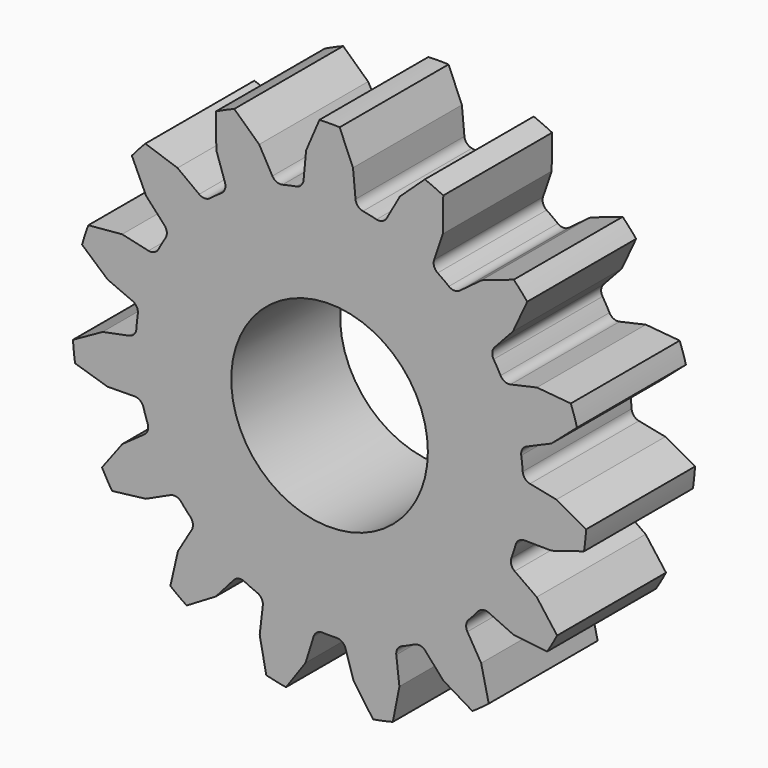
from build123d import *

# Parameters (mm, degrees)
F0_R     = 3.25
F1_DEPTH = 4.5


# Not quite as in the source:
# - ends of sketch curves that miss each other by under 0.0002 mm in the source are joined


with BuildPart() as f1:
    # F0 (on Front) → F1 (new body)
    with BuildSketch(Plane.XZ):
        with BuildLine():
            ThreePointArc((-6.3848473051, 0.378745021), (-6.458741388, 0.201395137), (-6.6250810223, 0.1052471112))
            Line((-6.6250810223, 0.1052471112), (-7.499995, -0.070416))
            Line((-7.499995, -0.070416), (-8.481787, -0.617539))
            ThreePointArc((-8.481787, -0.617539), (-8.4534361937, -0.9498951475), (-8.4120672698, -1.2808810391))
            Line((-8.4120672698, -1.2808810391), (-7.337975, -1.611925))
            Line((-7.337975, -1.611925), (-6.445659, -1.601845))
            ThreePointArc((-6.445659, -1.601845), (-6.2629631412, -1.6613077046), (-6.1538101366, -1.819419039))
            ThreePointArc((-6.1538101366, -1.819419039), (-6.0867618577, -2.039112292), (-6.0118718389, -2.2562609412))
            ThreePointArc((-6.0118718389, -2.2562609412), (-6.0072434399, -2.4483319562), (-6.120095855, -2.6038242044))
            Line((-6.120095855, -2.6038242044), (-6.84792, -3.12016))
            Line((-6.84792, -3.12016), (-7.522298, -4.019312))
            ThreePointArc((-7.522298, -4.019312), (-7.3612165371, -4.3114029523), (-7.1888002117, -4.5969471336))
            Line((-7.1888002117, -4.5969471336), (-6.07292, -4.462499))
            Line((-6.07292, -4.462499), (-5.261849, -4.090353))
            ThreePointArc((-5.261849, -4.090353), (-5.0707630565, -4.0703658396), (-4.9067374821, -4.1704104038))
            ThreePointArc((-4.9067374821, -4.1704104038), (-4.7561274158, -4.343839289), (-4.5993898038, -4.5117538102))
            ThreePointArc((-4.5993898038, -4.5117538102), (-4.5170386347, -4.6853377004), (-4.5568904277, -4.8732883391))
            Line((-4.5568904277, -4.8732883391), (-5.011778, -5.641017))
            Line((-5.011778, -5.641017), (-5.262135, -6.736727))
            ThreePointArc((-5.262135, -6.736727), (-4.9961722078, -6.9380502226), (-4.7225170454, -7.128782068))
            Line((-4.7225170454, -7.128782068), (-3.757802, -6.552084))
            Line((-3.757802, -6.552084), (-3.168217, -5.882218))
            ThreePointArc((-3.168217, -5.882218), (-3.0017803181, -5.7862379026), (-2.8112432041, -5.8109184175))
            ThreePointArc((-2.8112432041, -5.8109184175), (-2.6031126369, -5.9080957654), (-2.3916319825, -5.9977409564))
            ThreePointArc((-2.3916319825, -5.9977409564), (-2.2457975094, -6.1228225948), (-2.2057577098, -6.3107329173))
            Line((-2.2057577098, -6.3107329173), (-2.309055, -7.197108))
            Line((-2.309055, -7.197108), (-2.092101, -8.299918))
            ThreePointArc((-2.092101, -8.299918), (-1.7672462291, -8.3756592743), (-1.4396719873, -8.4385959262))
            Line((-1.4396719873, -8.4385959262), (-0.792926, -7.519371))
            Line((-0.792926, -7.519371), (-0.526772, -6.667613))
            ThreePointArc((-0.526772, -6.667613), (-0.4137637804, -6.5122339125), (-0.2296610073, -6.457282204))
            ThreePointArc((-0.2296610073, -6.457282204), (2.4984e-06, -6.461404), (0.229662, -6.457281998))
            ThreePointArc((0.229662, -6.457281998), (0.4137637804, -6.5122339125), (0.5267720218, -6.6676129932))
            Line((0.5267720218, -6.6676129932), (0.792926, -7.519371))
            Line((0.792926, -7.519371), (1.439676, -8.438595))
            ThreePointArc((1.439676, -8.438595), (1.7672522889, -8.3756579862), (2.0921050032, -8.2999170124))
            Line((2.0921050032, -8.2999170124), (2.309055, -7.197108))
            Line((2.309055, -7.197108), (2.205757, -6.310733))
            ThreePointArc((2.205757, -6.310733), (2.2457975094, -6.1228225948), (2.3916327595, -5.9977404031))
            ThreePointArc((2.3916327595, -5.9977404031), (2.6031159206, -5.9080943034), (2.8112438605, -5.8109177148))
            ThreePointArc((2.8112438605, -5.8109177148), (3.0017803181, -5.7862379026), (3.1682168748, -5.8822191102))
            Line((3.1682168748, -5.8822191102), (3.757802, -6.552084))
            Line((3.757802, -6.552084), (4.72252, -7.12878))
            ThreePointArc((4.72252, -7.12878), (4.9961769033, -6.9380468111), (5.2621377529, -6.7367246866))
            Line((5.2621377529, -6.7367246866), (5.011778, -5.641017))
            Line((5.011778, -5.641017), (4.556891, -4.873288))
            ThreePointArc((4.556891, -4.873288), (4.5170386766, -4.6853373435), (4.599391221, -4.5117522139))
            ThreePointArc((4.599391221, -4.5117522139), (4.7561281073, -4.3438385211), (4.9067371021, -4.1704100855))
            ThreePointArc((4.9067371021, -4.1704100855), (5.0707626825, -4.0703659239), (5.2618489304, -4.0903531516))
            Line((5.2618489304, -4.0903531516), (6.07292, -4.462499))
            Line((6.07292, -4.462499), (7.188798, -4.596951))
            ThreePointArc((7.188798, -4.596951), (7.361216975, -4.3114021938), (7.5222993001, -4.0193091579))
            Line((7.5222993001, -4.0193091579), (6.84792, -3.12016))
            Line((6.84792, -3.12016), (6.120096, -2.603824))
            ThreePointArc((6.120096, -2.603824), (6.0072434399, -2.4483319562), (6.0118725915, -2.2562588509))
            ThreePointArc((6.0118725915, -2.2562588509), (6.0867621941, -2.0391112566), (6.153810771, -1.8194179346))
            ThreePointArc((6.153810771, -1.8194179346), (6.2629631412, -1.6613077046), (6.4456589984, -1.6018451428))
            Line((6.4456589984, -1.6018451428), (7.337975, -1.611925))
            Line((7.337975, -1.611925), (8.412067, -1.280885))
            ThreePointArc((8.412067, -1.280885), (8.4534363514, -0.9498936467), (8.481787446, -0.6175350292))
            Line((8.481787446, -0.6175350292), (7.499995, -0.070416))
            Line((7.499995, -0.070416), (6.625082, 0.105247))
            ThreePointArc((6.625082, 0.105247), (6.4587417115, 0.2013947687), (6.3848473051, 0.378745021))
            ThreePointArc((6.3848473051, 0.378745021), (6.3649400086, 0.6075793237), (6.3368346677, 0.835549953))
            ThreePointArc((6.3368346677, 0.835549953), (6.3722414368, 1.0243877393), (6.5149571212, 1.1530187192))
            Line((6.5149571212, 1.1530187192), (7.334228, 1.506748))
            Line((7.334228, 1.506748), (8.180813, 2.246041))
            ThreePointArc((8.180813, 2.246041), (8.0839798549, 2.5652420945), (7.974697483, 2.8803981782))
            Line((7.974697483, 2.8803981782), (6.855252, 2.980885))
            Line((6.855252, 2.980885), (5.98453, 2.785503))
            ThreePointArc((5.98453, 2.785503), (5.7934636286, 2.8056817814), (5.6538228924, 2.9376439429))
            ThreePointArc((5.6538228924, 2.9376439429), (5.5425619412, 3.1385971137), (5.4241623811, 3.3354272386))
            ThreePointArc((5.4241623811, 3.3354272386), (5.3797004129, 3.5223406923), (5.4577587633, 3.697898218))
            Line((5.4577587633, 3.697898218), (6.062326, 4.354273))
            Line((6.062326, 4.354273), (6.535022, 5.373988))
            ThreePointArc((6.535022, 5.373988), (6.3167298633, 5.6262074349), (6.088709809, 5.8696678139))
            Line((6.088709809, 5.8696678139), (5.025173, 5.506148))
            Line((5.025173, 5.506148), (4.309199, 4.973502))
            ThreePointArc((4.309199, 4.973502), (4.1264437672, 4.9142226849), (3.9452018311, 4.9779787843))
            ThreePointArc((3.9452018311, 4.9779787843), (3.7618245482, 5.1163055389), (3.5736032135, 5.2479613173))
            ThreePointArc((3.5736032135, 5.2479613173), (3.4569607105, 5.4006300799), (3.4568644648, 5.5927591806))
            Line((3.4568644648, 5.5927591806), (3.742192, 6.438288))
            Line((3.742192, 6.438288), (3.759267, 7.562107))
            ThreePointArc((3.759267, 7.562107), (3.4572596135, 7.7037332148), (3.1499290285, 7.8334010714))
            Line((3.1499290285, 7.8334010714), (2.326197, 7.06873))
            Line((2.326197, 7.06873), (1.888768, 6.290921))
            ThreePointArc((1.888768, 6.290921), (1.7459243673, 6.1624334899), (1.554419964, 6.1469598562))
            ThreePointArc((1.554419964, 6.1469598562), (1.3306339934, 6.1987408207), (1.1051359772, 6.2424578697))
            ThreePointArc((1.1051359772, 6.2424578697), (0.9364810051, 6.3344853457), (0.8582472195, 6.5099649269))
            Line((0.8582472195, 6.5099649269), (0.775, 7.398447))
            Line((0.775, 7.398447), (0.3335, 8.432051))
            ThreePointArc((0.3335, 8.432051), (-1.4988e-06, 8.438596), (-0.3335029952, 8.4320508773))
            Line((-0.3335029952, 8.4320508773), (-0.775, 7.398447))
            Line((-0.775, 7.398447), (-0.858248, 6.509965))
            ThreePointArc((-0.858248, 6.509965), (-0.9364806674, 6.3344857115), (-1.1051359033, 6.2424574482))
            ThreePointArc((-1.1051359033, 6.2424574482), (-1.3306359057, 6.1987404142), (-1.5544199034, 6.146959614))
            ThreePointArc((-1.5544199034, 6.146959614), (-1.7459243673, 6.1624334899), (-1.8887681854, 6.2909208957))
            Line((-1.8887681854, 6.2909208957), (-2.326197, 7.06873))
            Line((-2.326197, 7.06873), (-3.149932, 7.8334))
            ThreePointArc((-3.149932, 7.8334), (-3.4572626886, 7.7037318457), (-3.759269185, 7.5621053752))
            Line((-3.759269185, 7.5621053752), (-3.742192, 6.438288))
            Line((-3.742192, 6.438288), (-3.456865, 5.59276))
            ThreePointArc((-3.456865, 5.59276), (-3.4569605775, 5.4006304728), (-3.5736028777, 5.2479608182))
            ThreePointArc((-3.5736028777, 5.2479608182), (-3.7618263316, 5.1163042431), (-3.9452020076, 4.9779790098))
            ThreePointArc((-3.9452020076, 4.9779790098), (-4.1264437672, 4.9142226849), (-4.3091988413, 4.9735022134))
            Line((-4.3091988413, 4.9735022134), (-5.025173, 5.506148))
            Line((-5.025173, 5.506148), (-6.088712, 5.869665))
            ThreePointArc((-6.088712, 5.869665), (-6.3167319914, 5.6262050713), (-6.5350238583, 5.3739858822))
            Line((-6.5350238583, 5.3739858822), (-6.062326, 4.354273))
            Line((-6.062326, 4.354273), (-5.457759, 3.697898))
            ThreePointArc((-5.457759, 3.697898), (-5.3797004129, 3.5223406923), (-5.4241620701, 3.3354270439))
            ThreePointArc((-5.4241620701, 3.3354270439), (-5.5425631892, 3.1385949521), (-5.6538231778, 2.9376430943))
            ThreePointArc((-5.6538231778, 2.9376430943), (-5.7934636286, 2.8056817814), (-5.9845300103, 2.785502954))
            Line((-5.9845300103, 2.785502954), (-6.855252, 2.980885))
            Line((-6.855252, 2.980885), (-7.974699, 2.880395))
            ThreePointArc((-7.974699, 2.880395), (-8.0839806406, 2.5652396762), (-8.1808133092, 2.2460390872))
            Line((-8.1808133092, 2.2460390872), (-7.334228, 1.506748))
            Line((-7.334228, 1.506748), (-6.514956, 1.153019))
            ThreePointArc((-6.514956, 1.153019), (-6.3722414368, 1.0243877393), (-6.3368349167, 0.8355489882))
            ThreePointArc((-6.3368349167, 0.8355489882), (-6.3649402163, 0.6075773468), (-6.3848473051, 0.378745021))
        make_face()
        with Locations((0, -0.061404)):
            Circle(F0_R, mode=Mode.SUBTRACT)
    extrude(amount=F1_DEPTH)


solid = f1.part
